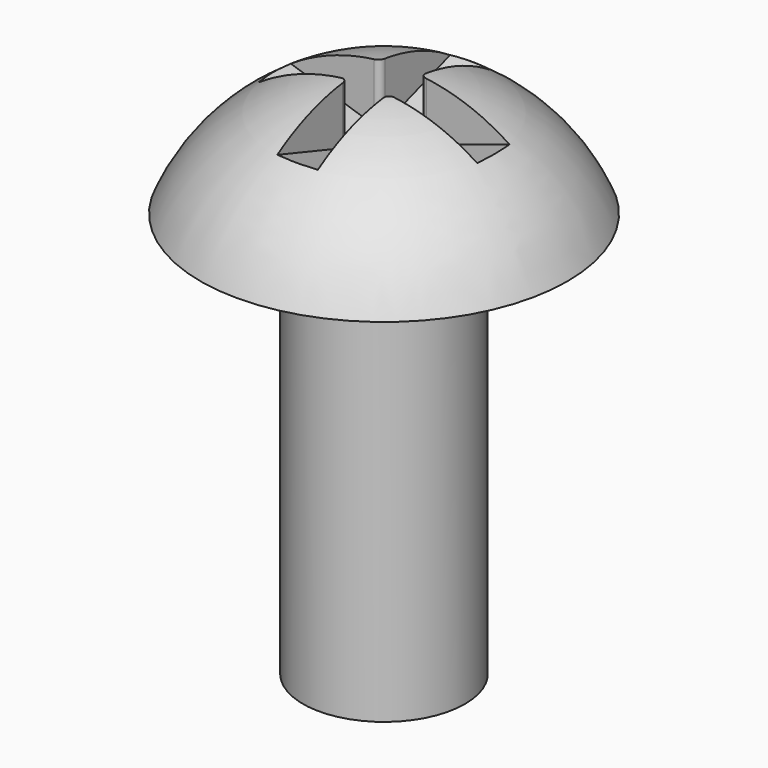
from build123d import *

# Parameters (mm, degrees)
F3_R           = 2
F4_DEPTH       = 10
F5_W           = 1
F5_H           = 0.8
F6_DEPTH       = 3
F6_DEPTH_BACK  = 3
F7_W           = 1
F7_H           = 0.8
F8_DEPTH       = 3
F8_DEPTH_BACK  = 3
F10_DEPTH      = 0.5
F10_DEPTH_BACK = 0.5
F11_T4_DEPTH   = 1
F12_T1_DEPTH   = 1
F13_T4_DEPTH   = 2.2322667456
F13_T10_DEPTH  = 1.8596499945
F13_T16_DEPTH  = 2.2322667452
F13_T22_DEPTH  = 1.859649995


# Not quite as in the source:
# - a fillet or chamfer that OpenCascade refuses, or shapes differently, is made with other operations: its cross-section is extruded or revolved along the edge and cut away or added


with BuildPart() as f2:
    # F0 (on Front) → F2 (revolve)
    with BuildSketch(Plane.XZ):
        with BuildLine():
            Line((0, 0), (0, 2.9999249461))
            ThreePointArc((0, 2.9999249461), (-2.7199502547, 2.1887322683), (-4.5270512497, 0))
            Line((-4.5270512497, 0), (0, 0))
        make_face()
    revolve(axis=Axis((0, 0, 1.5515517443), (0, 0, -1)))

    # F3 (on face) → F4 (join)
    with BuildSketch(Plane(origin=(0, 0, 0), x_dir=(1, 0, 0), z_dir=(0, 0, -1))):
        Circle(F3_R)
    extrude(amount=F4_DEPTH)

    # F5 (on Front) → F6 (cut, two sides)
    with BuildSketch(Plane.XZ) as f6_sk:
        with Locations((0, 2.6000668348)):
            Rectangle(F5_W, F5_H)
    extrude(amount=-F6_DEPTH, mode=Mode.SUBTRACT)
    extrude(f6_sk.sketch, amount=F6_DEPTH_BACK, mode=Mode.SUBTRACT)

    # F7 (on Right) → F8 (cut, two sides)
    with BuildSketch(Plane.YZ) as f8_sk:
        with Locations((0, 2.5815645484)):
            Rectangle(F7_W, F7_H)
    extrude(amount=F8_DEPTH, mode=Mode.SUBTRACT)
    extrude(f8_sk.sketch, amount=-F8_DEPTH_BACK, mode=Mode.SUBTRACT)

    # F9 (on Front) → F10 (cut, two sides)
    with BuildSketch(Plane.XZ) as f10_sk:
        Polygon((0.5315009621, 1.4676835854), (2.7381633418, 2.1851595957), (-2.7381633418, 2.1851595957), (-0.5315009621, 1.4676835854), (0, 1.4676835854), align=None)
    extrude(amount=F10_DEPTH, mode=Mode.SUBTRACT)
    extrude(f10_sk.sketch, amount=-F10_DEPTH_BACK, mode=Mode.SUBTRACT)

    # F11: chamfer of 0.733 x 2.18 on 1 edges, made by hand


with BuildPart() as f11_tool2:
    # F11_s3 → F11_t4 (new body)
    with BuildSketch(Plane.YZ.offset(0.5)):
        Polygon((2.68, 2.2000668348), (0.5, 1.4670668348), (0.5, 2.2000668348), align=None)
    extrude(amount=-F11_T4_DEPTH)

    split(bisect_by=Plane.XY.offset(1.4676835854), keep=Keep.TOP)


with BuildPart() as f2_1:
    add(f2.part)

    # F11_t1: cut F11_tool2
    add(f11_tool2.part, mode=Mode.SUBTRACT)

    # F12: chamfer of 2.183 x 0.73 on 1 edges, made by hand

    # F12_s2 → F12_t1 (cut)
    with BuildSketch(Plane.YZ.offset(-0.5)):
        Polygon((-0.5, 1.4700668348), (-2.683, 2.2000668348), (-0.5, 2.2000668348), align=None)
    extrude(amount=F12_T1_DEPTH, mode=Mode.SUBTRACT)

    # F13: fillet of radius 0.15 on 4 edges, made by hand


with BuildPart() as f13_tool2:
    # F13_s3 → F13_t4 (new body)
    with BuildSketch(Plane.XY.offset(3.3273335804)):
        with BuildLine():
            ThreePointArc((0.65, -0.5), (0.5439339828, -0.5439339828), (0.5, -0.65))
            Line((0.5, -0.65), (0.5, -0.5))
            Line((0.5, -0.5), (0.65, -0.5))
        make_face()
    extrude(amount=-F13_T4_DEPTH)

    split(bisect_by=Plane(origin=(-0.3807624945, 0, 1.1710694992), x_dir=(0, 1, 0), z_dir=(-0.309207193, 0, 0.950994696)), keep=Keep.TOP)

    split(bisect_by=Plane(origin=(0, 0.3918613388, 1.1718264421), x_dir=(1, 0, 0), z_dir=(0, 0.3171399402, 0.9483787526)), keep=Keep.TOP)


with BuildPart() as f2_2:
    add(f2_1.part)

    # F13_t1: cut F13_tool2
    add(f13_tool2.part, mode=Mode.SUBTRACT)


with BuildPart() as f13_tool8:
    # F13_s9 → F13_t10 (new body)
    with BuildSketch(Plane.XY.offset(3.3273335799)):
        with BuildLine():
            ThreePointArc((0.5, 0.65), (0.5439339828, 0.5439339828), (0.65, 0.5))
            Line((0.65, 0.5), (0.5, 0.5))
            Line((0.5, 0.5), (0.5, 0.65))
        make_face()
    extrude(amount=-F13_T10_DEPTH)

    split(bisect_by=Plane(origin=(0, -0.3923936318, 1.16700971), x_dir=(1, 0, 0), z_dir=(0, -0.3187050207, 0.9478539496)), keep=Keep.TOP)

    split(bisect_by=Plane(origin=(-0.3807624945, 0, 1.1710694992), x_dir=(0, 1, 0), z_dir=(-0.309207193, 0, 0.950994696)), keep=Keep.TOP)


with BuildPart() as f2_3:
    add(f2_2.part)

    # F13_t7: cut F13_tool8
    add(f13_tool8.part, mode=Mode.SUBTRACT)


with BuildPart() as f13_tool14:
    # F13_s15 → F13_t16 (new body)
    with BuildSketch(Plane.XY.offset(1.0950668348)):
        with BuildLine():
            ThreePointArc((-0.65, -0.5), (-0.5439339828, -0.5439339828), (-0.5, -0.65))
            Line((-0.5, -0.65), (-0.5, -0.5))
            Line((-0.5, -0.5), (-0.65, -0.5))
        make_face()
    extrude(amount=F13_T16_DEPTH)

    split(bisect_by=Plane(origin=(0.3807624945, 0, 1.1710694992), x_dir=(0, 1, 0), z_dir=(0.309207193, 0, 0.950994696)), keep=Keep.TOP)

    split(bisect_by=Plane(origin=(0, 0.3918613388, 1.1718264421), x_dir=(1, 0, 0), z_dir=(0, 0.3171399402, 0.9483787526)), keep=Keep.TOP)


with BuildPart() as f2_4:
    add(f2_3.part)

    # F13_t13: cut F13_tool14
    add(f13_tool14.part, mode=Mode.SUBTRACT)


with BuildPart() as f13_tool20:
    # F13_s21 → F13_t22 (new body)
    with BuildSketch(Plane.XY.offset(3.3273335804)):
        with BuildLine():
            ThreePointArc((-0.65, 0.5), (-0.5439339828, 0.5439339828), (-0.5, 0.65))
            Line((-0.5, 0.65), (-0.5, 0.5))
            Line((-0.5, 0.5), (-0.65, 0.5))
        make_face()
    extrude(amount=-F13_T22_DEPTH)

    split(bisect_by=Plane(origin=(0.3807624945, 0, 1.1710694992), x_dir=(0, 1, 0), z_dir=(0.309207193, 0, 0.950994696)), keep=Keep.TOP)

    split(bisect_by=Plane(origin=(0, -0.3923936318, 1.16700971), x_dir=(1, 0, 0), z_dir=(0, -0.3187050207, 0.9478539496)), keep=Keep.TOP)


with BuildPart() as f2_5:
    add(f2_4.part)

    # F13_t19: cut F13_tool20
    add(f13_tool20.part, mode=Mode.SUBTRACT)


solid = f2_5.part
